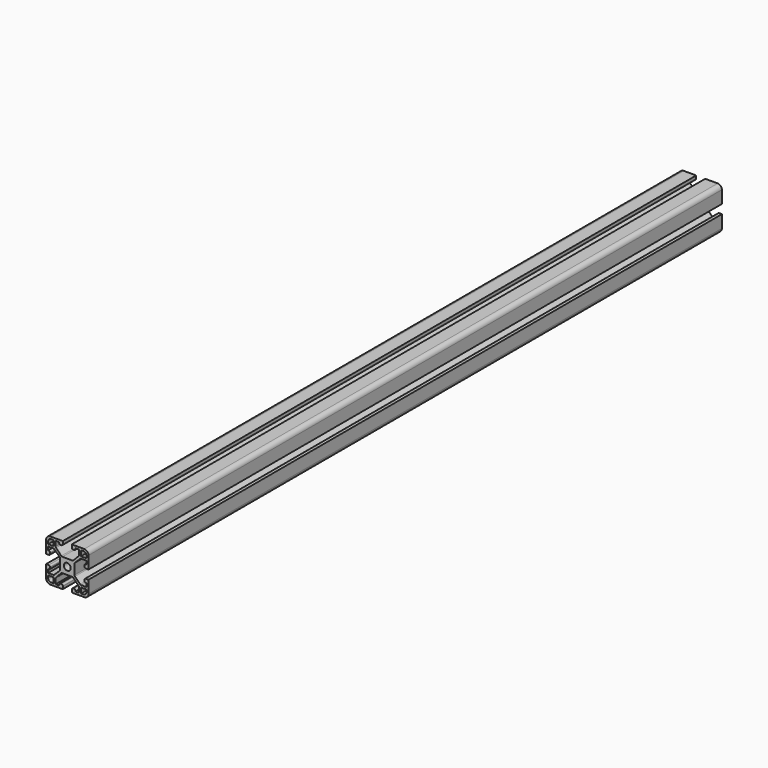
from build123d import *

# Parameters (mm, degrees)
F0_R     = 2.45
F1_DEPTH = 460
F2_DEPTH = 100


# Not quite as in the source:
# - ends of sketch curves that miss each other by under 0.0002 mm in the source are joined


with BuildPart() as f1:
    # F0 (on Front) → F1 (new body)
    with BuildSketch(Plane.XZ):
        with BuildLine():
            Line((-3.1749674082, 15), (-12, 15))
            ThreePointArc((-12, 15), (-14.1213203436, 14.1213203436), (-15, 12))
            Line((-15, 12), (-15, 3.175))
            Line((-15, 3.175), (-13.0855346263, 3.175))
            ThreePointArc((-13.0855346263, 3.175), (-12.3835980145, 3.4627605788), (-12.0856407741, 4.1604300138))
            Line((-12.0856407741, 4.1604300138), (-12.0761692778, 4.8104300138))
            ThreePointArc((-12.0761692778, 4.8104300138), (-12.3638237087, 5.5269366118), (-13.0760631299, 5.825))
            Line((-13.0760631299, 5.825), (-13.5, 5.825))
            Line((-13.5, 5.825), (-13.5, 8.225))
            Line((-13.5, 8.225), (-9.8968845016, 8.225))
            ThreePointArc((-9.8968845016, 8.225), (-9.5279915195, 8.1544718757), (-9.2111331975, 7.9528359354))
            Line((-9.2111331975, 7.9528359354), (-5.4142486959, 4.3754933338))
            ThreePointArc((-5.4142486959, 4.3754933338), (-5.1819174045, 4.0440465354), (-5.1, 3.6476573984))
            Line((-5.1, 3.6476573984), (-5.1, -3.4999243287))
            ThreePointArc((-5.1, -3.4999243287), (-5.1782354607, -3.8876744211), (-5.4007002683, -4.2147528992))
            Line((-5.4007002683, -4.2147528992), (-9.2084959767, -7.9398285705))
            ThreePointArc((-9.2084959767, -7.9398285705), (-9.5301904718, -8.1509666761), (-9.9077957084, -8.225))
            Line((-9.9077957084, -8.225), (-13.5, -8.225))
            Line((-13.5, -8.225), (-13.5, -5.825))
            Line((-13.5, -5.825), (-13.0760631299, -5.825))
            ThreePointArc((-13.0760631299, -5.825), (-12.3638237087, -5.5269366118), (-12.0761692778, -4.8104300138))
            Line((-12.0761692778, -4.8104300138), (-12.0856407741, -4.1604300138))
            ThreePointArc((-12.0856407741, -4.1604300138), (-12.3835980145, -3.4627605788), (-13.0855346263, -3.175))
            Line((-13.0855346263, -3.175), (-15, -3.175))
            Line((-15, -3.175), (-15, -12))
            ThreePointArc((-15, -12), (-14.1213203436, -14.1213203436), (-12, -15))
            Line((-12, -15), (-3.175, -15))
            Line((-3.175, -15), (-3.175, -13.0855346263))
            ThreePointArc((-3.175, -13.0855346263), (-3.4627605788, -12.3835980145), (-4.1604300138, -12.0856407741))
            Line((-4.1604300138, -12.0856407741), (-4.8104300138, -12.0761692778))
            ThreePointArc((-4.8104300138, -12.0761692778), (-5.5269366118, -12.3638237087), (-5.825, -13.0760631299))
            Line((-5.825, -13.0760631299), (-5.825, -13.5))
            Line((-5.825, -13.5), (-8.225, -13.5))
            Line((-8.225, -13.5), (-8.225, -9.8968845016))
            ThreePointArc((-8.225, -9.8968845016), (-8.1544718757, -9.5279915195), (-7.9528359354, -9.2111331975))
            Line((-7.9528359354, -9.2111331975), (-4.3754933338, -5.4142486959))
            ThreePointArc((-4.3754933338, -5.4142486959), (-4.0440465354, -5.1819174045), (-3.6476573984, -5.1))
            Line((-3.6476573984, -5.1), (3.4999243287, -5.1))
            ThreePointArc((3.4999243287, -5.1), (3.8876744211, -5.1782354607), (4.2147528992, -5.4007002683))
            Line((4.2147528992, -5.4007002683), (7.9398285705, -9.2084959767))
            ThreePointArc((7.9398285705, -9.2084959767), (8.1509666761, -9.5301904718), (8.225, -9.9077957084))
            Line((8.225, -9.9077957084), (8.225, -13.5))
            Line((8.225, -13.5), (5.825, -13.5))
            Line((5.825, -13.5), (5.825, -13.0760631299))
            ThreePointArc((5.825, -13.0760631299), (5.5269366118, -12.3638237087), (4.8104300138, -12.0761692778))
            Line((4.8104300138, -12.0761692778), (4.1604300138, -12.0856407741))
            ThreePointArc((4.1604300138, -12.0856407741), (3.4627605788, -12.3835980145), (3.175, -13.0855346263))
            Line((3.175, -13.0855346263), (3.175, -15))
            Line((3.175, -15), (12, -15))
            ThreePointArc((12, -15), (14.1213203436, -14.1213203436), (15, -12))
            Line((15, -12), (15, -3.175))
            Line((15, -3.175), (13.0855346263, -3.175))
            ThreePointArc((13.0855346263, -3.175), (12.3835980145, -3.4627605788), (12.0856407741, -4.1604300138))
            Line((12.0856407741, -4.1604300138), (12.0761692778, -4.8104300138))
            ThreePointArc((12.0761692778, -4.8104300138), (12.3638237087, -5.5269366118), (13.0760631299, -5.825))
            Line((13.0760631299, -5.825), (13.5, -5.825))
            Line((13.5, -5.825), (13.5, -8.225))
            Line((13.5, -8.225), (9.9077957084, -8.225))
            ThreePointArc((9.9077957084, -8.225), (9.5301904718, -8.1509666761), (9.2084959767, -7.9398285705))
            Line((9.2084959767, -7.9398285705), (5.4007002683, -4.2147528992))
            ThreePointArc((5.4007002683, -4.2147528992), (5.1782354607, -3.8876744211), (5.1, -3.4999243287))
            Line((5.1, -3.4999243287), (5.1, 3.6476573984))
            ThreePointArc((5.1, 3.6476573984), (5.1819174045, 4.0440465354), (5.4142486959, 4.3754933338))
            Line((5.4142486959, 4.3754933338), (9.2111331975, 7.9528359354))
            ThreePointArc((9.2111331975, 7.9528359354), (9.5279915195, 8.1544718757), (9.8968845016, 8.225))
            Line((9.8968845016, 8.225), (13.5, 8.225))
            Line((13.5, 8.225), (13.5, 5.825))
            Line((13.5, 5.825), (13.0760631299, 5.825))
            ThreePointArc((13.0760631299, 5.825), (12.3638237087, 5.5269366118), (12.0761692778, 4.8104300138))
            Line((12.0761692778, 4.8104300138), (12.0856407741, 4.1604300138))
            ThreePointArc((12.0856407741, 4.1604300138), (12.3835980145, 3.4627605788), (13.0855346263, 3.175))
            Line((13.0855346263, 3.175), (15, 3.175))
            Line((15, 3.175), (15, 12))
            ThreePointArc((15, 12), (14.1213203436, 14.1213203436), (12, 15))
            Line((12, 15), (3.1750325918, 15))
            Line((3.1750325918, 15), (3.1750325918, 13.0854824722))
            ThreePointArc((3.1750325918, 13.0854824722), (3.4627931706, 12.3835458604), (4.1604626057, 12.0855886201))
            Line((4.1604626057, 12.0855886201), (4.8104626057, 12.0761171237))
            ThreePointArc((4.8104626057, 12.0761171237), (5.5269692036, 12.3637715546), (5.8250325918, 13.0760109758))
            Line((5.8250325918, 13.0760109758), (5.8250325918, 13.4999478459))
            Line((5.8250325918, 13.4999478459), (8.2250325918, 13.4999478459))
            Line((8.2250325918, 13.4999478459), (8.2250325918, 9.8968323476))
            ThreePointArc((8.2250325918, 9.8968323476), (8.1545044675, 9.5279393654), (7.9528685272, 9.2110810434))
            Line((7.9528685272, 9.2110810434), (4.3755259256, 5.4141965418))
            ThreePointArc((4.3755259256, 5.4141965418), (4.0440791272, 5.1818652505), (3.6476899902, 5.0999478459))
            Line((3.6476899902, 5.0999478459), (-3.4998917369, 5.0999478459))
            ThreePointArc((-3.4998917369, 5.0999478459), (-3.8876418293, 5.1781833067), (-4.2147203074, 5.4006481142))
            Line((-4.2147203074, 5.4006481142), (-7.9397959787, 9.2084438226))
            ThreePointArc((-7.9397959787, 9.2084438226), (-8.1509340843, 9.5301383177), (-8.2249674082, 9.9077435543))
            Line((-8.2249674082, 9.9077435543), (-8.2249674082, 13.4999478459))
            Line((-8.2249674082, 13.4999478459), (-5.8249674082, 13.4999478459))
            Line((-5.8249674082, 13.4999478459), (-5.8249674082, 13.0760109758))
            ThreePointArc((-5.8249674082, 13.0760109758), (-5.5269040199, 12.3637715546), (-4.810397422, 12.0761171237))
            Line((-4.810397422, 12.0761171237), (-4.160397422, 12.0855886201))
            ThreePointArc((-4.160397422, 12.0855886201), (-3.462727987, 12.3835458604), (-3.1749674082, 13.0854824722))
            Line((-3.1749674082, 13.0854824722), (-3.1749674082, 15))
        make_face()
        with BuildLine():
            Line((-13.5, -11.5), (-13.5, -9.7))
            Line((-13.5, -9.7), (-9.7, -9.7))
            Line((-9.7, -9.7), (-9.7, -13.5))
            Line((-9.7, -13.5), (-11.5, -13.5))
            ThreePointArc((-11.5, -13.5), (-12.9142135624, -12.9142135624), (-13.5, -11.5))
        make_face(mode=Mode.SUBTRACT)
        with BuildLine():
            Line((9.7, -9.7), (13.5, -9.7))
            Line((13.5, -9.7), (13.5, -11.5))
            ThreePointArc((13.5, -11.5), (12.9142135624, -12.9142135624), (11.5, -13.5))
            Line((11.5, -13.5), (9.7, -13.5))
            Line((9.7, -13.5), (9.7, -9.7))
        make_face(mode=Mode.SUBTRACT)
        with BuildLine():
            ThreePointArc((-13.5, 11.5), (-12.9142135624, 12.9142135624), (-11.5, 13.5))
            Line((-11.5, 13.5), (-9.7, 13.5))
            Line((-9.7, 13.5), (-9.7, 9.7))
            Line((-9.7, 9.7), (-13.5, 9.7))
            Line((-13.5, 9.7), (-13.5, 11.5))
        make_face(mode=Mode.SUBTRACT)
        Circle(F0_R, mode=Mode.SUBTRACT)
        with BuildLine():
            Line((9.7, 13.5), (11.5, 13.5))
            ThreePointArc((11.5, 13.5), (12.9142135624, 12.9142135624), (13.5, 11.5))
            Line((13.5, 11.5), (13.5, 9.7))
            Line((13.5, 9.7), (9.7, 9.7))
            Line((9.7, 9.7), (9.7, 13.5))
        make_face(mode=Mode.SUBTRACT)
    extrude(amount=F1_DEPTH)

    # F2 (add): a face of the model
    f2_faces = [f1.faces().sort_by_distance(p)[0] for p in [
        (5.2291627207, -460, 12.6659491494),
    ]]
    extrude(f2_faces, amount=F2_DEPTH)


solid = f1.part
